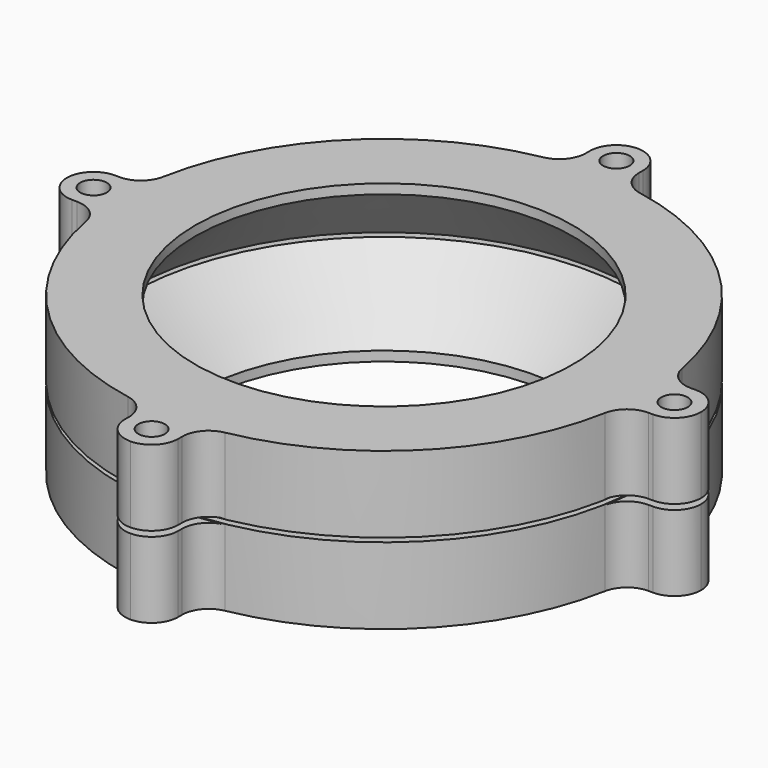
from build123d import *

# Parameters (mm, degrees)
F3_DEPTH          = 57
F4_R              = 19.99999
F7_ANGLE          = 180
F10_D             = 20
F10_CBORE_D       = 25
F10_CBORE_DEPTH   = 10
F10_2_D           = 20
F10_2_CBORE_D     = 25
F10_2_CBORE_DEPTH = 10


# Not quite as in the source:
# - a fillet or chamfer is up to 0.001 mm smaller than in the source, because OpenCascade refuses the exact size


with BuildPart() as f1:
    # F0 (on Front) → F1 (revolve)
    with BuildSketch(Plane.XZ):
        Polygon((-122.6969882846, 61.8426688015), (-114.2994761467, 61.8426688015), (-66.1537349224, 112.0411325246), (-66.1537349224, 119.318977464), (-122.6969882846, 119.318977464), align=None)
    revolve(axis=Axis((75.8012831211, 0, 61.6655610502), (0, 0, 1)))

    # F2 (on face) → F3 (join)
    with BuildSketch(Plane.XY.offset(119.318977464)):
        with BuildLine():
            ThreePointArc((-121.6868526011, -20), (-122.4442935194, -10.0127465525), (-122.6969882846, 0))
            Line((-122.6969882846, 0), (-162.6969882846, 0))
            Line((-162.6969882846, 0), (-162.6969882846, -20))
            Line((-162.6969882846, -20), (-121.6868526011, -20))
        make_face()
        with BuildLine():
            Line((-162.6969882846, 0), (-122.6969882846, 0))
            ThreePointArc((-122.6969882846, 0), (-122.4442935194, 10.0127465525), (-121.6868526011, 20))
            Line((-121.6868526011, 20), (-162.6969882846, 20))
            Line((-162.6969882846, 20), (-162.6969882846, 0))
        make_face()
        with BuildLine():
            ThreePointArc((55.8012831211, 197.4881357222), (65.7885365686, 198.2455766405), (75.8012831211, 198.4982714057))
            Line((75.8012831211, 198.4982714057), (75.8012831211, 238.4982714057))
            Line((75.8012831211, 238.4982714057), (55.8012831211, 238.4982714057))
            Line((55.8012831211, 238.4982714057), (55.8012831211, 197.4881357223))
        make_face()
        with BuildLine():
            Line((75.8012831211, 238.4982714057), (75.8012831211, 198.4982714057))
            ThreePointArc((75.8012831211, 198.4982714057), (85.8140296736, 198.2455766405), (95.8012831211, 197.4881357222))
            Line((95.8012831211, 197.4881357222), (95.8012831211, 238.4982714057))
            Line((95.8012831211, 238.4982714057), (75.8012831211, 238.4982714057))
        make_face()
        with BuildLine():
            Line((75.8012831211, -238.4982714057), (75.8012831211, -198.4982714057))
            ThreePointArc((75.8012831211, -198.4982714057), (65.7885365686, -198.2455766405), (55.8012831211, -197.4881357222))
            Line((55.8012831211, -197.4881357222), (55.8012831211, -238.4982714057))
            Line((55.8012831211, -238.4982714057), (75.8012831211, -238.4982714057))
        make_face()
        with BuildLine():
            ThreePointArc((95.8012831211, -197.4881357223), (85.8140296736, -198.2455766405), (75.8012831211, -198.4982714057))
            Line((75.8012831211, -198.4982714057), (75.8012831211, -238.4982714057))
            Line((75.8012831211, -238.4982714057), (95.8012831211, -238.4982714057))
            Line((95.8012831211, -238.4982714057), (95.8012831211, -197.4881357223))
        make_face()
        with BuildLine():
            Line((314.2995545268, 0), (274.2995545268, 0))
            ThreePointArc((274.2995545268, 0), (274.0468597616, -10.0127465525), (273.2894188434, -20))
            Line((273.2894188434, -20), (314.2995545268, -20))
            Line((314.2995545268, -20), (314.2995545268, 0))
        make_face()
        with BuildLine():
            ThreePointArc((273.2894188434, 20), (274.0468597616, 10.0127465525), (274.2995545268, 0))
            Line((274.2995545268, 0), (314.2995545268, 0))
            Line((314.2995545268, 0), (314.2995545268, 20))
            Line((314.2995545268, 20), (273.2894188434, 20))
        make_face()
    extrude(amount=-F3_DEPTH)

    # F4 (radius 20 in the source; OpenCascade refuses exactly that, so slightly less here)
    f4_edges = [f1.edges().sort_by_distance(p)[0] for p in [
        (95.801283, -197.488136, 90.818977),
        (55.801283, -197.488136, 90.818977),
        (273.289419, -20, 90.818977),
        (-121.686853, 20, 90.818977),
        (95.801283, 197.488136, 90.818977),
        (55.801283, 197.488136, 90.818977),
        (273.289419, 20, 90.818977),
        (-121.686853, -20, 90.818977),
        (-162.696988, -20, 90.818977),
        (-162.696988, 20, 90.818977),
        (55.801283, 238.498271, 90.818977),
        (95.801283, 238.498271, 90.818977),
        (314.299555, 20, 90.818977),
        (314.299555, -20, 90.818977),
        (95.801283, -238.498271, 90.818977),
        (55.801283, -238.498271, 90.818977),
    ]]
    fillet(f4_edges, radius=F4_R)


with BuildPart() as f1b:
    # F0 (on Front) → F1, piece 2 (revolve)
    with BuildSketch(Plane.XZ):
        Polygon((-114.2994761467, 61.4884532988), (-122.6969882846, 61.4884532988), (-122.6969882846, 4.0121446364), (-66.1537349224, 4.0121446364), (-66.1537349224, 11.2899895757), align=None)
    revolve(axis=Axis((75.8012831211, 0, 61.6655610502), (0, 0, 1)))


with BuildPart() as f6_1:
    # F6: copy of F1
    add(f1.part.moved(Location((0, 0, -59))))

    # F10#2 (through all)
    with Locations(Plane(origin=(0, 0, -57.681022536), x_dir=(1, 0, 0), z_dir=(0, 0, -1))):
        with Locations((75.8012831211, 218.4982714057), (-142.6969882846, 0), (75.8012831211, -218.4982714057), (294.2995545268, 0)):
            CounterBoreHole(F10_2_D / 2, F10_2_CBORE_D / 2, F10_2_CBORE_DEPTH)


with BuildPart() as f1_1:
    # F7: moved
    add(f1.part.rotate(Axis((75.8012831211, 0, 119.318977464), (0, -1, 0)), F7_ANGLE))


with BuildPart() as f1_2:
    # F8: moved
    add(f1_1.part.moved(Location((0, 0, -177))))

    # F10 (through all)
    with Locations(Plane(origin=(0, 0, -57.681022536), x_dir=(1, 0, 0), z_dir=(0, 0, -1))):
        with Locations((75.8012831211, 218.4982714057), (-142.6969882846, 0), (75.8012831211, -218.4982714057), (294.2995545268, 0)):
            CounterBoreHole(F10_D / 2, F10_CBORE_D / 2, F10_CBORE_DEPTH)


solid = Compound([f6_1.part, f1_2.part])
